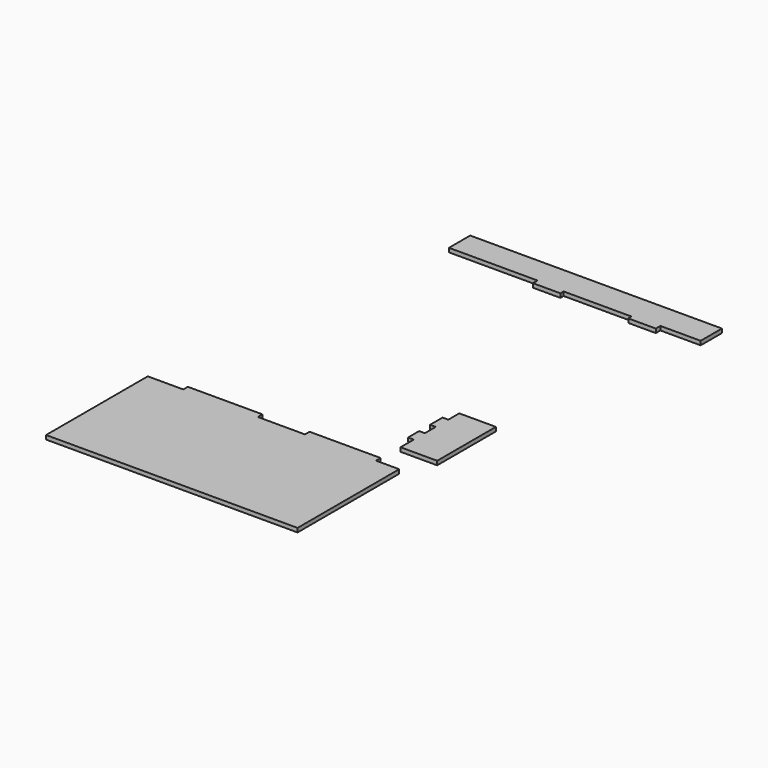
from build123d import *

# Parameters (mm, degrees)
F1_DEPTH = 4.45


# Not quite as in the source:
# - a feature names something its author has since deleted; it is built from what else it names


with BuildPart() as f1:
    # F0 (on Top) → F1 (new body)
    with BuildSketch(Plane.XY):
        Polygon((-1.7402413478, -299.4968297958), (-40.9429369935, -299.4968297958), (-40.9429369935, -439.7566318512), (236.5724275148, -439.7566318512), (236.5724275148, -299.4968297958), (215.0616164281, -299.4968297958), (210.8597586522, -299.4968297958), (210.8597586522, -293.1668297958), (132.5597586522, -293.1668297958), (132.5597586522, -299.4968297958), (80.5597586522, -299.4968297958), (80.5597586522, -293.1668297958), (-1.7402413478, -293.1668297958), align=None)
    extrude(amount=F1_DEPTH)


with BuildPart() as f1b:
    # F0 (on Top) → F1, piece 2 (new body)
    with BuildSketch(Plane.XY):
        Polygon((252.2649765015, -185.7516178083), (211.8477205402, -185.7516178083), (211.8477205402, -200.6451304226), (211.8477205402, -200.8938822837), (205.5177205402, -200.8938822837), (205.5177205402, -218.1938822837), (211.8477205402, -218.1938822837), (211.8477205402, -226.2631509995), (211.8477205402, -230.1938822837), (211.8477205402, -232.7680322837), (211.8477205402, -233.1938822837), (205.5161595345, -233.1938822837), (205.5161595345, -248.4938822837), (211.8477205402, -248.4938822837), (211.8477205402, -266.7746841908), (252.2649765015, -266.7746841908), align=None)
    extrude(amount=F1_DEPTH)


with BuildPart() as f1c:
    # F0 (on Top) → F1, piece 3 (new body)
    with BuildSketch(Plane.XY):
        Polygon((109.6645991251, 49.936733744), (109.6645991251, 43.606733744), (139.9645991251, 43.606733744), (139.9645991251, 48.056733744), (214.9645991251, 48.056733744), (214.9645991251, 43.606733744), (245.2645991251, 43.606733744), (245.2645991251, 49.936733744), (289.7008654758, 49.936733744), (289.7008654758, 79.2557150126), (11.8996296078, 79.2557150126), (11.8996296078, 49.936733744), (86.1305896078, 49.936733744), align=None)
    extrude(amount=F1_DEPTH)


solid = Compound([f1.part, f1b.part, f1c.part])
